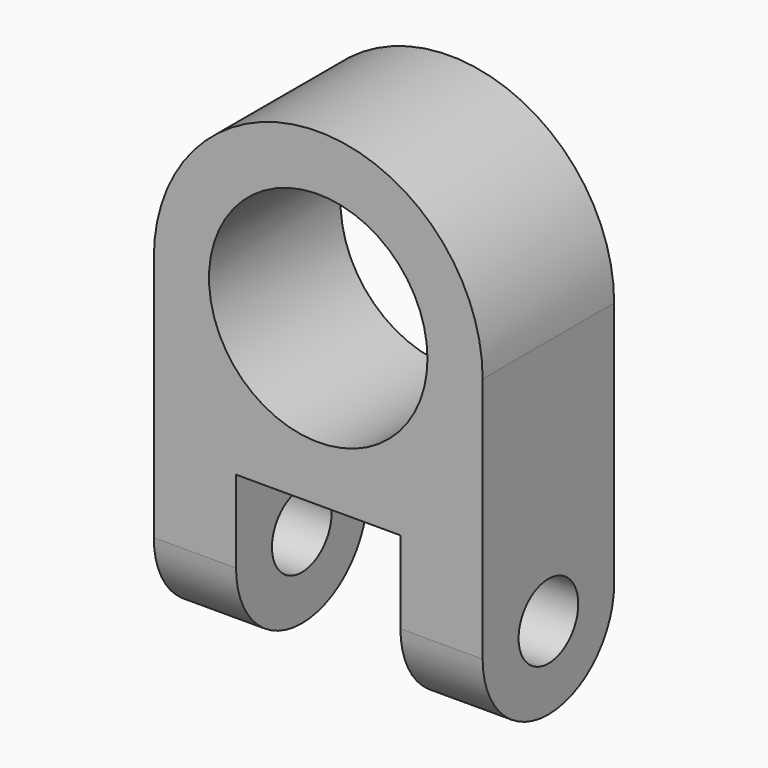
from build123d import *

# Parameters (mm, degrees)
F0_R     = 8.4375
F1_DEPTH = 12.7
F2_R     = 6.34999
F3_R     = 2.88125
F4_DEPTH = 25.401


# Not quite as in the source:
# - a fillet or chamfer is up to 0.001 mm smaller than in the source, because OpenCascade refuses the exact size


with BuildPart() as f1:
    # F0 (on Front) → F1 (new body)
    with BuildSketch(Plane.XZ):
        with BuildLine():
            ThreePointArc((0, -12.7), (-8.9802561211, -8.9802561211), (-12.7, 0))
            Line((-12.7, 0), (-12.7, -25.4))
            Line((-12.7, -25.4), (-6.35, -25.4))
            Line((-6.35, -25.4), (-6.35, -12.7))
            Line((-6.35, -12.7), (0, -12.7))
        make_face()
        with BuildLine():
            Line((12.7, -25.4), (12.7, 0))
            ThreePointArc((12.7, 0), (8.9802561211, -8.9802561211), (0, -12.7))
            Line((0, -12.7), (6.35, -12.7))
            Line((6.35, -12.7), (6.35, -25.4))
            Line((6.35, -25.4), (12.7, -25.4))
        make_face()
        with BuildLine():
            ThreePointArc((0, -12.7), (8.9802561211, -8.9802561211), (12.7, 0))
            ThreePointArc((12.7, 0), (0, 12.7), (-12.7, 0))
            ThreePointArc((-12.7, 0), (-8.9802561211, -8.9802561211), (0, -12.7))
        make_face()
        Circle(F0_R, mode=Mode.SUBTRACT)
    extrude(amount=F1_DEPTH)

    # F2 (radius 6.35 in the source; OpenCascade refuses exactly that, so slightly less here)
    f2_edges = [f1.edges().sort_by_distance(p)[0] for p in [
        (-9.525, -12.7, -25.4),
        (-9.525, 0, -25.4),
        (9.525, -12.7, -25.4),
        (9.525, 0, -25.4),
    ]]
    fillet(f2_edges, radius=F2_R)

    # F3 (on face) → F4 (cut, through all)
    with BuildSketch(Plane.YZ.offset(12.7)):
        with Locations((-6.35, -19.05)):
            Circle(F3_R)
    extrude(amount=-F4_DEPTH, mode=Mode.SUBTRACT)


solid = f1.part
